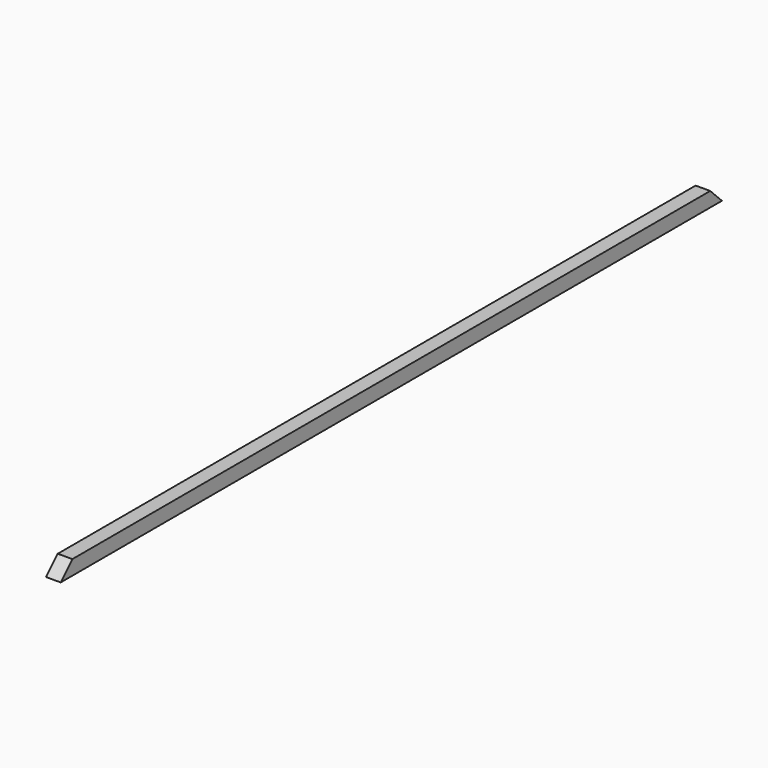
from build123d import *

# Parameters (mm, degrees)
F0_W     = 3.81
F0_H     = 215.519
F1_DEPTH = 3.81
F2_SIZE  = 3.80999
F3_SIZE  = 3.80999


# Not quite as in the source:
# - a fillet or chamfer is up to 0.001 mm smaller than in the source, because OpenCascade refuses the exact size


with BuildPart() as f1:
    # F0 (on Top) → F1 (new body)
    with BuildSketch(Plane.XY):
        with Locations((88.7727327645, 106.5352801529)):
            Rectangle(F0_W, F0_H)
    extrude(amount=F1_DEPTH)

    # F2 (size 3.81 in the source; OpenCascade refuses exactly that, so slightly less here)
    f2_edges = [f1.edges().sort_by_distance(p)[0] for p in [
        (88.772733, -1.22422, 3.81),
    ]]
    chamfer(f2_edges, length=F2_SIZE)

    # F3 (size 3.81 in the source; OpenCascade refuses exactly that, so slightly less here)
    f3_edges = [f1.edges().sort_by_distance(p)[0] for p in [
        (88.772733, 214.29478, 3.81),
    ]]
    chamfer(f3_edges, length=F3_SIZE)


solid = f1.part
